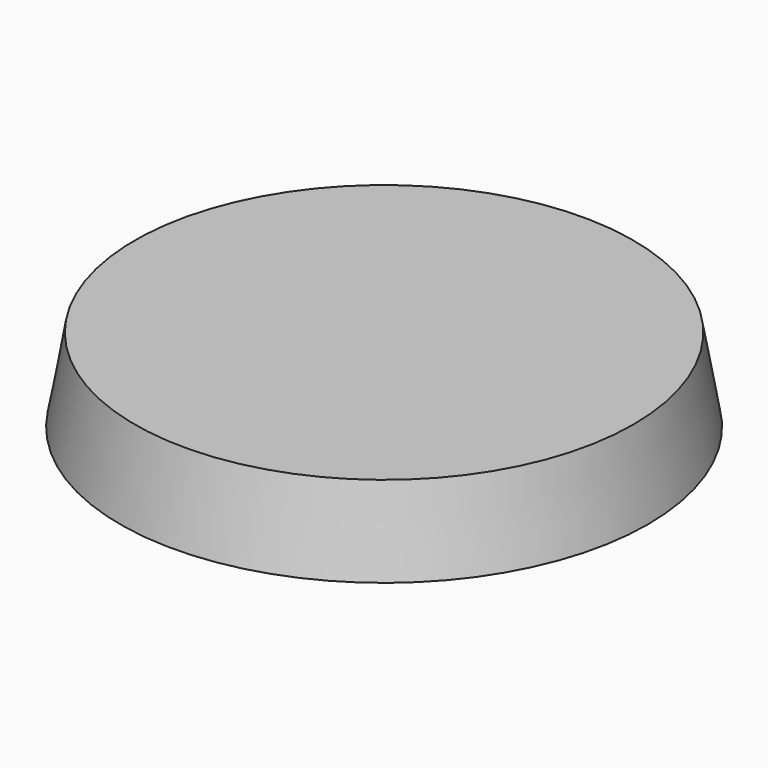
from build123d import *

# Parameters (mm, degrees)
F0_R         = 30
F1_DEPTH     = 10
F1_TAPER     = -10
F2_TEXT_SIZE = 21.7763698228
F3_DEPTH     = 1


# Not quite as in the source:
# - Text() gives the source's letters only with a copy of the font that has no kerning and outlines rounded to 1/6400 em; it was checked with that copy


with BuildPart() as f1:
    # F0 (on Top) → F1 (new body)
    with BuildSketch(Plane.XY):
        Circle(F0_R)
    extrude(amount=-F1_DEPTH, taper=F1_TAPER)

    # F2 (on face) → F3 (cut)
    with BuildSketch(Plane(origin=(0, 0, -10), x_dir=(1, 0, 0), z_dir=(0, 0, -1))):
        with Locations((-29, -4.6789862724)):
            Text('Maria', F2_TEXT_SIZE, font='Open Sans', font_style=FontStyle.ITALIC, text_align=(TextAlign.LEFT, TextAlign.BOTTOM))
    extrude(amount=-F3_DEPTH, mode=Mode.SUBTRACT)


solid = f1.part
